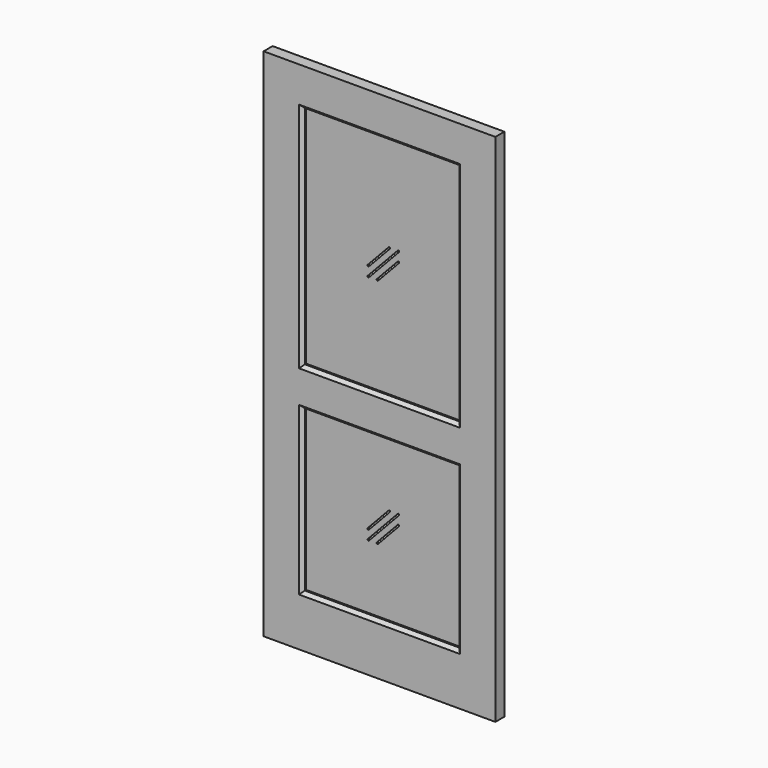
from build123d import *

# Parameters (mm, degrees)
F0_W          = 914.4
F0_H          = 2032
F0_W_2        = 609.6
F0_H_2        = 633.4125
F0_H_3        = 890.5875
F1_DEPTH      = 22.225
F1_DEPTH_BACK = 22.225
F2_W          = 609.6
F2_H          = 890.5875
F2_H_2        = 633.4125
F3_DEPTH      = 3.175
F3_DEPTH_BACK = 3.175
F4_SIZE       = 12.7


# Not quite as in the source:
# - a length typed as a fraction of an inch, garbled in the dataset ("3 / 203.2 mm" for 3/8 in), is restored


with BuildPart() as f1:
    # F0 (on Front) → F1 (new body, two sides)
    with BuildSketch(Plane.XZ) as f1_sk:
        with Locations((457.2, 1016)):
            Rectangle(F0_W, F0_H)
        with Locations((457.2, 519.90625)):
            Rectangle(F0_W_2, F0_H_2, mode=Mode.SUBTRACT)
        with Locations((457.2, 1434.30625)):
            Rectangle(F0_W_2, F0_H_3, mode=Mode.SUBTRACT)
    extrude(amount=F1_DEPTH)
    extrude(f1_sk.sketch, amount=-F1_DEPTH_BACK)

    # F2 (on Front) → F3 (join, two sides)
    with BuildSketch(Plane.XZ) as f3_sk:
        with Locations((457.2, 1434.30625)):
            Rectangle(F2_W, F2_H)
        with BuildLine():
            Line((395.6148101771, 1373.3735846555), (514.1566101771, 1499.5861846555))
            ThreePointArc((514.1566101771, 1499.5861846555), (518.6445346555, 1499.7268398229), (518.7851898229, 1495.2389153445))
            Line((518.7851898229, 1495.2389153445), (400.2433898229, 1369.0263153445))
            ThreePointArc((400.2433898229, 1369.0263153445), (395.7554653445, 1368.8856601771), (395.6148101771, 1373.3735846555))
        make_face(mode=Mode.SUBTRACT)
        with BuildLine():
            Line((395.6148101771, 1411.4735846555), (478.3722068767, 1499.5861846555))
            ThreePointArc((478.3722068767, 1499.5861846555), (482.8601313551, 1499.7268398229), (483.0007865224, 1495.2389153445))
            Line((483.0007865224, 1495.2389153445), (400.2433898229, 1407.1263153445))
            ThreePointArc((400.2433898229, 1407.1263153445), (395.7554653445, 1406.9856601771), (395.6148101771, 1411.4735846555))
        make_face(mode=Mode.SUBTRACT)
        with BuildLine():
            Line((431.3992134776, 1373.3735846555), (514.1566101771, 1461.4861846555))
            ThreePointArc((514.1566101771, 1461.4861846555), (518.6445346555, 1461.6268398229), (518.7851898229, 1457.1389153445))
            Line((518.7851898229, 1457.1389153445), (436.0277931233, 1369.0263153445))
            ThreePointArc((436.0277931233, 1369.0263153445), (431.5398686449, 1368.8856601771), (431.3992134776, 1373.3735846555))
        make_face(mode=Mode.SUBTRACT)
        with Locations((457.2, 519.90625)):
            Rectangle(F2_W, F2_H_2)
        with BuildLine():
            Line((395.6148101771, 497.0735846555), (478.3722068767, 585.1861846555))
            ThreePointArc((478.3722068767, 585.1861846555), (482.8601313551, 585.3268398229), (483.0007865224, 580.8389153445))
            Line((483.0007865224, 580.8389153445), (400.2433898229, 492.7263153445))
            ThreePointArc((400.2433898229, 492.7263153445), (395.7554653445, 492.5856601771), (395.6148101771, 497.0735846555))
        make_face(mode=Mode.SUBTRACT)
        with BuildLine():
            Line((395.6148101771, 458.9735846555), (514.1566101771, 585.1861846555))
            ThreePointArc((514.1566101771, 585.1861846555), (518.6445346555, 585.3268398229), (518.7851898229, 580.8389153445))
            Line((518.7851898229, 580.8389153445), (400.2433898229, 454.6263153445))
            ThreePointArc((400.2433898229, 454.6263153445), (395.7554653445, 454.4856601771), (395.6148101771, 458.9735846555))
        make_face(mode=Mode.SUBTRACT)
        with BuildLine():
            Line((431.3992134776, 458.9735846555), (514.1566101771, 547.0861846555))
            ThreePointArc((514.1566101771, 547.0861846555), (518.6445346555, 547.2268398229), (518.7851898229, 542.7389153445))
            Line((518.7851898229, 542.7389153445), (436.0277931233, 454.6263153445))
            ThreePointArc((436.0277931233, 454.6263153445), (431.5398686449, 454.4856601771), (431.3992134776, 458.9735846555))
        make_face(mode=Mode.SUBTRACT)
    extrude(amount=F3_DEPTH)
    extrude(f3_sk.sketch, amount=-F3_DEPTH_BACK)

    # F4
    f4_edges = [f1.edges().sort_by_distance(p)[0] for p in [
        (457.2, -22.225, 1879.6),
        (762, -22.225, 1434.30625),
        (457.2, -22.225, 989.0125),
        (152.4, -22.225, 1434.30625),
        (457.2, -22.225, 836.6125),
        (152.4, -22.225, 519.90625),
        (762, -22.225, 519.90625),
        (457.2, -22.225, 203.2),
        (457.2, 22.225, 836.6125),
        (762, 22.225, 519.90625),
        (152.4, 22.225, 519.90625),
        (457.2, 22.225, 203.2),
        (152.4, 22.225, 1434.30625),
        (457.2, 22.225, 989.0125),
        (762, 22.225, 1434.30625),
        (457.2, 22.225, 1879.6),
    ]]
    chamfer(f4_edges, length=F4_SIZE)


solid = f1.part
